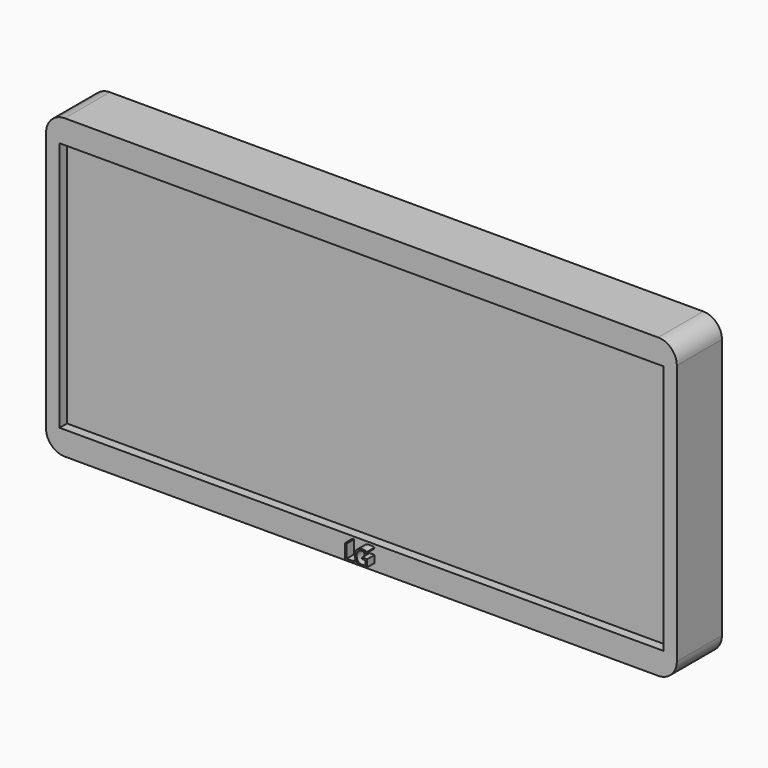
from build123d import *

# Parameters (mm, degrees)
F0_W         = 168.9975213834
F0_H         = 79.8070542514
F1_DEPTH     = 15.1
F2_W         = 161.7281883955
F2_H         = 67.1224817634
F3_DEPTH     = 2.5
F4_TEXT_SIZE = 5.537411198
F5_DEPTH     = 2.5
F6_R         = 5


# Not quite as in the source:
# - Text() gives the source's letters only with a copy of the font that has no kerning and outlines rounded to 1/6400 em; it was checked with that copy


with BuildPart() as f1:
    # F0 (on Front) → F1 (new body)
    with BuildSketch(Plane.XZ):
        Rectangle(F0_W, F0_H)
    extrude(amount=F1_DEPTH)

    # F2 (on face) → F3 (cut)
    with BuildSketch(Plane.XZ.offset(15.1)):
        Rectangle(F2_W, F2_H)
    extrude(amount=-F3_DEPTH, mode=Mode.SUBTRACT)

    # F4 (on face) → F5 (join)
    with BuildSketch(Plane.XZ.offset(15.1)):
        with Locations((-2.9753580457, -38.1703600287)):
            Text('LG', F4_TEXT_SIZE, font='Open Sans', text_align=(TextAlign.LEFT, TextAlign.BOTTOM))
    extrude(amount=F5_DEPTH)

    # F6
    f6_edges = [f1.edges().sort_by_distance(p)[0] for p in [
        (-84.498761, -7.55, 39.903527),
        (-84.498761, -7.55, -39.903527),
        (84.498761, -7.55, 39.903527),
        (84.498761, -7.55, -39.903527),
    ]]
    fillet(f6_edges, radius=F6_R)


solid = f1.part
